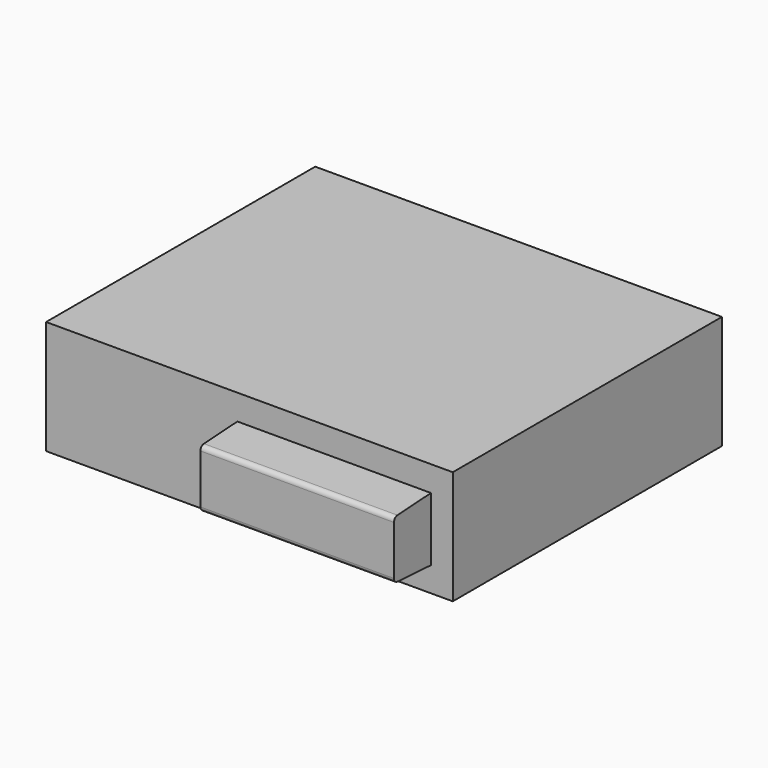
from build123d import *

# Parameters (mm, degrees)
F0_W       = 440
F0_H       = 123
F1_DEPTH   = 364
F2_R       = 40
F3_DEPTH   = 25
F4_W       = 209.3812078238
F4_H       = 68.7625966966
F5_DEPTH   = 50
F6_SIZE2   = 2.99999
F6_SIZE    = 49.99999
F6_2_SIZE2 = 2.99999
F6_2_SIZE  = 49.99999
F7_R       = 5


# Not quite as in the source:
# - a fillet or chamfer is up to 0.001 mm smaller than in the source, because OpenCascade refuses the exact size


with BuildPart() as f1:
    # F0 (on Front) → F1 (new body)
    with BuildSketch(Plane.XZ):
        Rectangle(F0_W, F0_H)
    extrude(amount=F1_DEPTH)

    # F2 (on face) → F3 (join)
    with BuildSketch(Plane(origin=(0, 0, 0), x_dir=(-1, 0, 0), z_dir=(0, 1, 0))):
        with Locations((-160, 0)):
            Circle(F2_R)
        with Locations((160, 0)):
            Circle(F2_R)
    extrude(amount=F3_DEPTH)

    # F4 (on face) → F5 (join)
    with BuildSketch(Plane.XZ.offset(364)):
        with Locations((91.689683497, -0.3388542682)):
            Rectangle(F4_W, F4_H)
    extrude(amount=F5_DEPTH)

    # F6 (size 50 and 3 in the source; OpenCascade refuses exactly that, so slightly less here)
    f6_edges = [f1.edges().sort_by_distance(p)[0] for p in [
        (91.689683, -414, 34.042444),
    ]]
    f6_side = f1.faces().sort_by_distance((91.689683, -389, 34.042444))[0]
    chamfer(f6_edges, length=F6_SIZE, length2=F6_SIZE2, reference=f6_side)

    # F6#2 (size 50 and 3 in the source; OpenCascade refuses exactly that, so slightly less here)
    f6_2_edges = [f1.edges().sort_by_distance(p)[0] for p in [
        (91.689683, -414, -34.720153),
    ]]
    f6_2_side = f1.faces().sort_by_distance((91.689683, -389, -34.720153))[0]
    chamfer(f6_2_edges, length=F6_2_SIZE, length2=F6_2_SIZE2, reference=f6_2_side)

    # F7
    f7_edges = [f1.edges().sort_by_distance(p)[0] for p in [
        (91.689683, -414, 31.042454),
        (91.689683, -414, -31.720163),
    ]]
    fillet(f7_edges, radius=F7_R)


solid = f1.part
